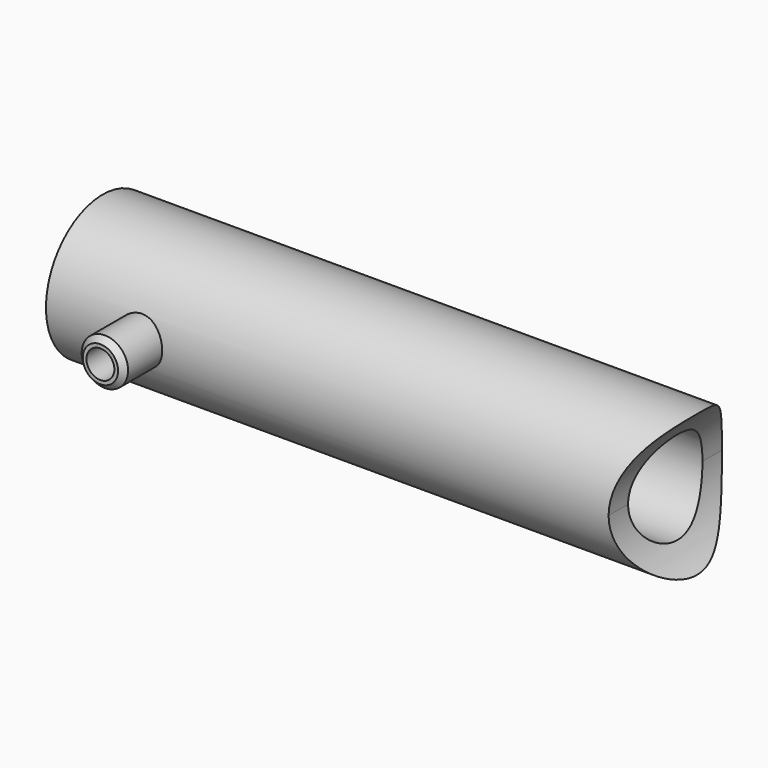
from build123d import *
from build123d import SkipClean  # not in build123d's __all__

# Parameters (mm, degrees)
F0_R      = 12.5
F0_R_2    = 7.5
F1_DEPTH  = 64
F2_R      = 38.1
F2_R_2    = 25
F3_DEPTH  = 100
F4_DEPTH  = 50
F5_SIZE   = 3
F6_R      = 25
F7_DEPTH  = 200
F8_R      = 7.5
F9_DEPTH  = 50
F10_DEPTH = 100
F11_R     = 7.5
F12_DEPTH = 50
F13_DEPTH = 75


with BuildPart() as f1:
    # F0 (on Front) → F1 (new body)
    with BuildSketch(Plane.XZ):
        Circle(F0_R)
        Circle(F0_R_2, mode=Mode.SUBTRACT)
    extrude(amount=F1_DEPTH)

    # F2 (on Right) → F3 (join)
    with BuildSketch(Plane.YZ):
        Circle(F2_R)
        Circle(F2_R_2, mode=Mode.SUBTRACT)
    extrude(amount=F3_DEPTH)

    # F2 (on Right) → F4 (join)
    with BuildSketch(Plane.YZ):
        Circle(F2_R)
        Circle(F2_R_2, mode=Mode.SUBTRACT)
    extrude(amount=-F4_DEPTH)

    # F5
    f5_edges = [f1.edges().sort_by_distance(p)[0] for p in [
        (-12.5, -64, 0),
    ]]
    chamfer(f5_edges, length=F5_SIZE)

    # F6 (on face) → F7 (cut)
    with BuildSketch(Plane(origin=(-50, 0, 0), x_dir=(0, -1, 0), z_dir=(-1, 0, 0))):
        Circle(F6_R)
    extrude(amount=-F7_DEPTH, mode=Mode.SUBTRACT)

    # F8 (on face) → F9 (cut)
    with BuildSketch(Plane.XZ.offset(64)):
        Circle(F8_R)
    extrude(amount=-F9_DEPTH, mode=Mode.SUBTRACT)

    # F10 (add): a face of the model
    f10_faces = [f1.faces().sort_by_distance(p)[0] for p in [
        (100, -37.0223692655, 0),
    ]]
    with SkipClean():  # cleaning this boolean's faces spoils the solid; the shape is the same uncleaned
        extrude(f10_faces, amount=F10_DEPTH)

    # F11 (on face) → F12 (cut)
    with BuildSketch(Plane.XZ.offset(64)):
        Circle(F11_R)
    with SkipClean():  # cleaning this boolean's faces spoils the solid; the shape is the same uncleaned
        extrude(amount=-F12_DEPTH, mode=Mode.SUBTRACT)

    # F13 (add): a face of the model
    f13_faces = [f1.faces().sort_by_distance(p)[0] for p in [
        (200, -37.0223692655, 0),
    ]]
    extrude(f13_faces, amount=F13_DEPTH)

    # F14 (on Top) → F15 (revolve, cut)
    with BuildSketch(Plane.XY):
        Polygon((280.1408666709, 52.4849742776), (252.6145875454, 51.9348941743), (252.6145875454, -50.6588555872), (280.1408666709, -51.4342445287), align=None)
    with SkipClean():  # cleaning this boolean's faces spoils the solid; the shape is the same uncleaned
        revolve(axis=Axis((303.6976158619, 0.4289562068, 0), (0, -1, 0)), mode=Mode.SUBTRACT)


solid = f1.part
